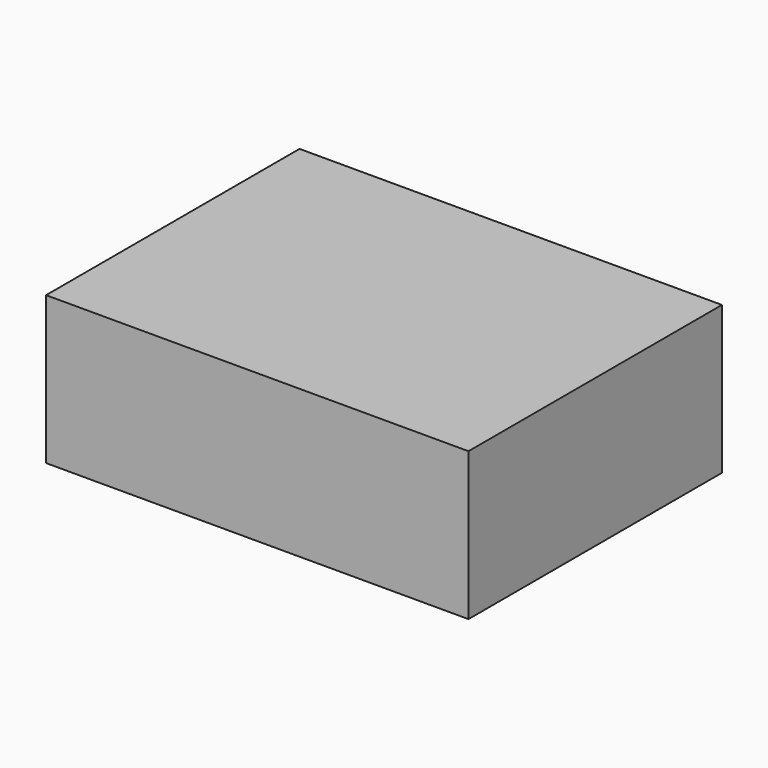
from build123d import *

# Parameters (mm, degrees)
F0_W     = 20
F0_H     = 15
F1_DEPTH = 7
F3_W     = 10.6
F3_H     = 10.6
F4_DEPTH = 3.6
F5_R     = 2.2
F6_DEPTH = 7


with BuildPart() as f1:
    # F0 (on Top) → F1 (new body)
    with BuildSketch(Plane.XY):
        Rectangle(F0_W, F0_H)
    extrude(amount=F1_DEPTH)

    # F3 (on offset) → F4 (cut)
    with BuildSketch(Plane.XY.offset(2)):
        with Locations((-5, 0)):
            Rectangle(F3_W, F3_H)
    extrude(amount=F4_DEPTH, mode=Mode.SUBTRACT)

    # F5 (on Top) → F6 (join, through all)
    with BuildSketch(Plane.XY):
        with Locations((-5, 0)):
            Circle(F5_R)
    extrude(amount=F6_DEPTH)


solid = f1.part
